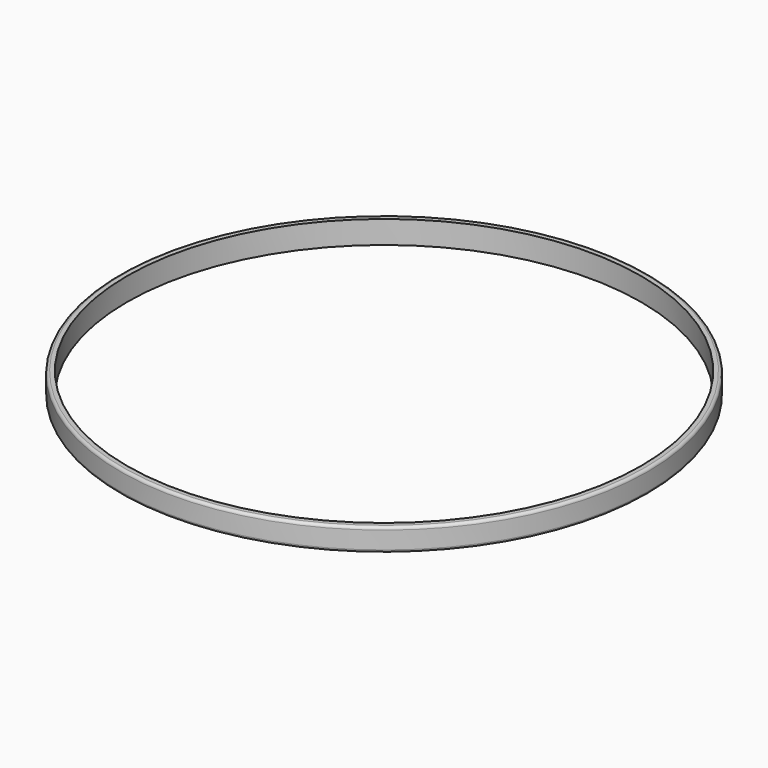
from build123d import *


# Not quite as in the source:
# - the program builds the solid bodies; features that only make, move or delete a surface that nothing else refers to are left out


with BuildPart() as f3:
    # F2 (on Front) → F3 (revolve)
    with BuildSketch(Plane.XZ):
        with BuildLine():
            Line((71.2252706289, -0.9149015559), (71.2252706289, -7.2649015559))
            Line((71.2252706289, -7.2649015559), (72.3682706289, -7.2649015559))
            ThreePointArc((72.3682706289, -7.2649015559), (72.9070859962, -7.0417169231), (73.1302706289, -6.5029015559))
            Line((73.1302706289, -6.5029015559), (73.1302706289, -1.6769015559))
            ThreePointArc((73.1302706289, -1.6769015559), (72.9070859962, -1.1380861886), (72.3682706289, -0.9149015559))
            Line((72.3682706289, -0.9149015559), (71.2252706289, -0.9149015559))
        make_face()
    revolve(axis=Axis((0, 0, -37.46373), (0, 0, -1)))


solid = f3.part
